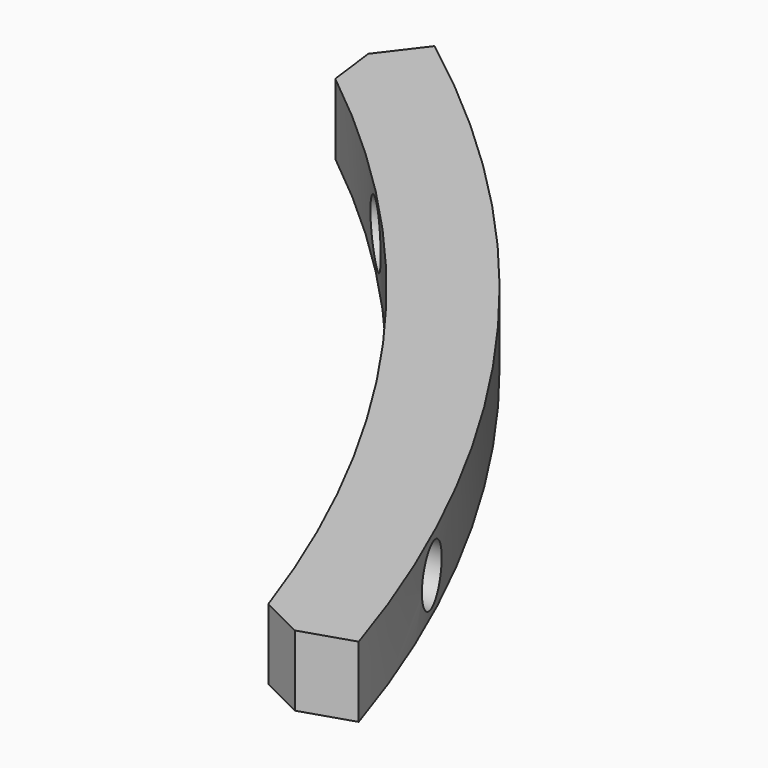
from build123d import *

# Parameters (mm, degrees)
F1_DEPTH    = 4
F4_D        = 3.2
F5_T1_DEPTH = 14.1810362517


# Not quite as in the source:
# - a fillet or chamfer that OpenCascade refuses, or shapes differently, is made with other operations: its cross-section is extruded or revolved along the edge and cut away or added


with BuildPart() as f1:
    # F0 (on Top) → F1 (new body)
    with BuildSketch(Plane.XY):
        with BuildLine():
            ThreePointArc((54.4209333808, 71.682368892), (73.4574706888, 52), (85.6943365292, 27.5041939859))
            Line((85.6943365292, 27.5041939859), (90.4551330031, 29.0322047629))
            ThreePointArc((90.4551330031, 29.0322047629), (77.5384412827, 54.8888888889), (57.4443185686, 75.6647227193))
            Line((57.4443185686, 75.6647227193), (54.4209333808, 71.682368892))
        make_face()
    extrude(amount=F1_DEPTH)

    # F4 (through all)
    with Locations(Plane.YZ.offset(90.457)):
        with Locations((39.0287227929, 1.9947474357), (63.0079358816, 2.0034648478)):
            Hole(F4_D / 2)

    # F5: chamfer of 2 on 2 edges, made by hand

    # F5_s2 → F5_t1 (cut)
    with BuildSketch(Plane.XY.offset(-5.0905181258)):
        with BuildLine():
            Line((87.5779535576, 28.1087539864), (85.0761677414, 29.3606144765))
            ThreePointArc((85.0761677414, 29.3606144765), (85.3813536757, 28.4609283843), (85.6943365292, 27.5041939859))
            Line((85.6943365292, 27.5041939859), (87.5779535576, 28.1087539864))
        make_face()
        with BuildLine():
            Line((55.6171407495, 73.2579937949), (55.9663848396, 70.4823649432))
            ThreePointArc((55.9663848396, 70.4823649432), (55.2192662472, 71.0692101766), (54.4209333808, 71.682368892))
            Line((54.4209333808, 71.682368892), (55.6171407495, 73.2579937949))
        make_face()
    extrude(amount=F5_T1_DEPTH, mode=Mode.SUBTRACT)


solid = f1.part
